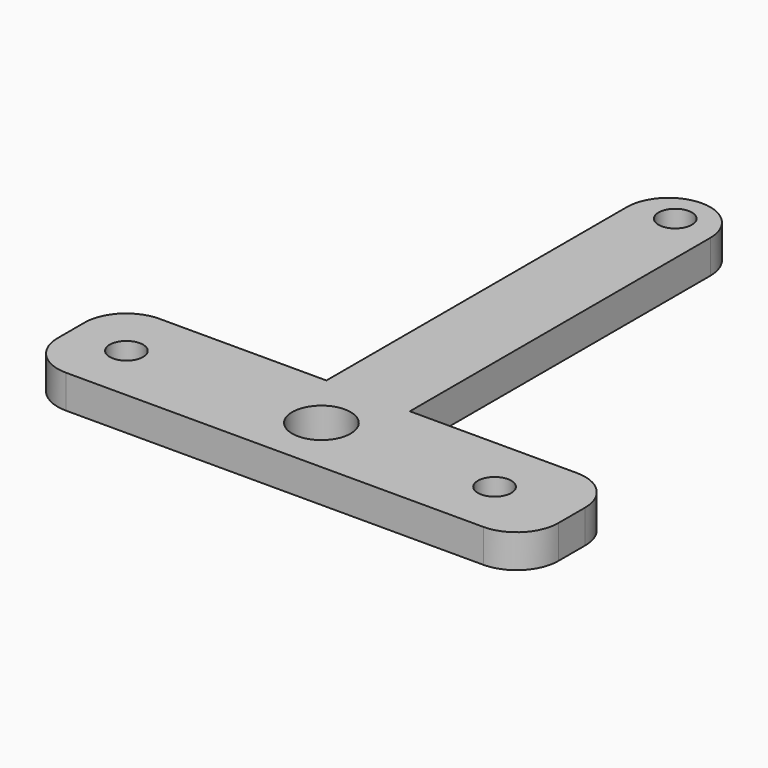
from build123d import *

# Parameters (mm, degrees)
F1_DEPTH = 4
F2_R     = 2
F2_R_2   = 3.5
F3_DEPTH = 25
F4_R     = 4.99999


# Not quite as in the source:
# - a fillet or chamfer is up to 0.001 mm smaller than in the source, because OpenCascade refuses the exact size


with BuildPart() as f1:
    # F0 (on Top) → F1 (new body)
    with BuildSketch(Plane.XY):
        Polygon((-5, 0), (-30, 0), (-30, -14), (30, -14), (30, 0), (5, 0), (5, 50), (-5, 50), align=None)
    extrude(amount=F1_DEPTH)

    # F2 (on face) → F3 (cut)
    with BuildSketch(Plane.XY.offset(4)):
        with Locations((-23.3714003116, -7)):
            Circle(F2_R)
        with Locations((20.7536797971, -7)):
            Circle(F2_R)
        with Locations((0, -7)):
            Circle(F2_R_2)
        with Locations((0, 46)):
            Circle(F2_R)
    extrude(amount=-F3_DEPTH, mode=Mode.SUBTRACT)

    # F4 (radius 5 in the source; OpenCascade refuses exactly that, so slightly less here)
    f4_edges = [f1.edges().sort_by_distance(p)[0] for p in [
        (-5, 50, 2),
        (5, 50, 2),
        (30, 0, 2),
        (30, -14, 2),
        (-30, -14, 2),
        (-30, 0, 2),
    ]]
    fillet(f4_edges, radius=F4_R)


solid = f1.part
